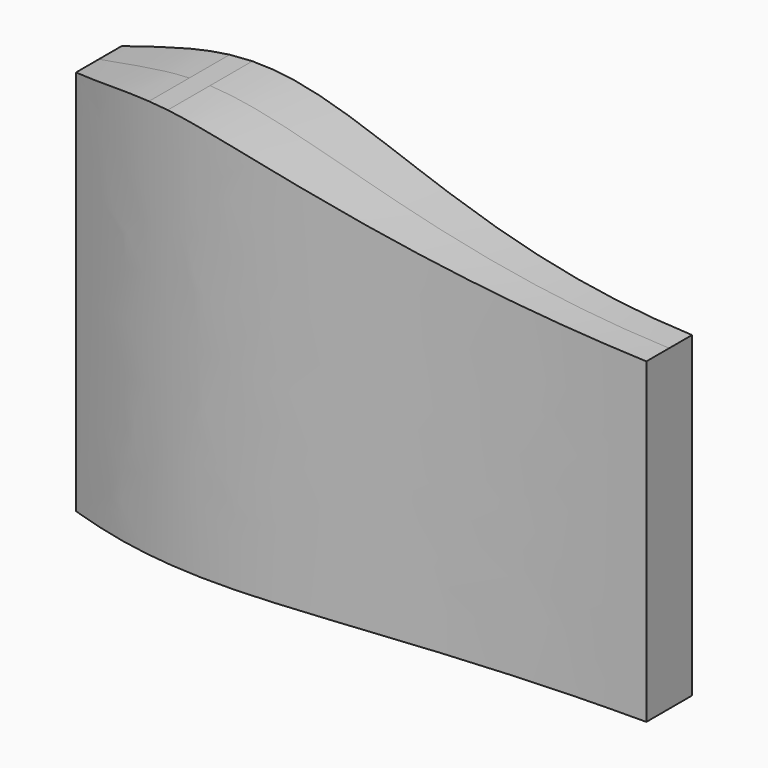
from build123d import *

# Parameters (mm, degrees)
F1_DEPTH      = 2133.6
F3_DEPTH      = 543.38083
F3_DEPTH_BACK = 650.61769


with BuildPart() as f1:
    # F0 (on Top) → F1 (new body)
    with BuildSketch(Plane.XY):
        with BuildLine():
            add(Edge.make_bspline(
                [(-1524, 152.4), (-1219.2, 254), (-522.232182492, 371.7581676674), (533.4, 154.0921661663), (1524, 152.4)],
                knots=[0, 0, 0, 0, 0.3968086679, 1, 1, 1, 1], degree=3))
            Line((-1524, 152.4), (-1524, -152.4))
            add(Edge.make_bspline(
                [(-1524, -152.4), (-1219.2, -254), (-522.232182492, -372.3147623717), (533.4, -152.4), (1524, -152.4)],
                knots=[0, 0, 0, 0, 0.3968086679, 1, 1, 1, 1], degree=3))
            Line((1524, -152.4), (1524, 152.4))
        make_face()
    extrude(amount=F1_DEPTH)

    # F2 (on Front) → F3 (cut, two sides)
    with BuildSketch(Plane.XZ) as f3_sk:
        with BuildLine():
            Line((-1905, 2553.8010597229), (-1905, 2032))
            add(Edge.make_bspline(
                [(-1905, 2032), (-1549.4, 2021.84), (-798.7639864346, 2359.1821919655), (366.4164065367, 1691.64), (1778, 1691.64)],
                knots=[0, 0, 0, 0, 0.3741653136, 1, 1, 1, 1], degree=3))
            Line((1778, 1691.64), (1777.6815891266, 2553.8010597229))
            Line((1777.6815891266, 2553.8010597229), (-1905, 2553.8010597229))
        make_face()
    extrude(amount=-F3_DEPTH, mode=Mode.SUBTRACT)
    extrude(f3_sk.sketch, amount=F3_DEPTH_BACK, mode=Mode.SUBTRACT)


solid = f1.part
